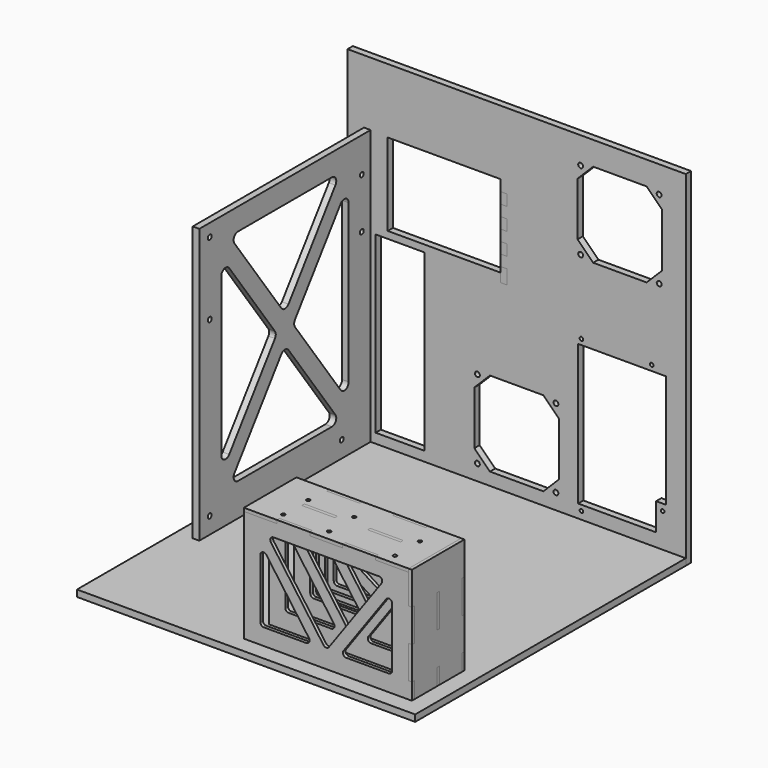
from build123d import *

# Parameters (mm, degrees)
F1_DEPTH  = 6
F3_DEPTH  = 6
F7_DEPTH  = 6
F10_D     = 4.4
F11_R     = 5
F12_W     = 44.5
F12_H     = 159
F12_W_2   = 102.7
F12_H_2   = 74.93
F13_DEPTH = 314.001
F15_W     = 22
F15_H     = 82.93
F16_DEPTH = 6
F17_W     = 6
F17_H     = 10
F18_DEPTH = 145.301
F21_DEPTH = 314.001
F22_D     = 3.3
F24_DEPTH = 314.001
F25_D     = 4.4
F27_W     = 153
F27_H     = 111
F28_DEPTH = 3
F29_W     = 30
F29_H     = 6
F29_H_2   = 3
F29_W_2   = 3
F29_H_3   = 30
F30_DEPTH = 315.001
F31_R     = 3
F35_W     = 150
F35_H     = 59.8
F36_DEPTH = 3
F38_D     = 3.3
F39_W     = 59.8
F39_H     = 105
F40_DEPTH = 3
F43_W     = 103
F43_H     = 79
F44_DEPTH = 3
F45_W     = 20
F45_H     = 6
F45_W_2   = 3
F45_H_2   = 2
F45_H_3   = 13
F45_H_4   = 3
F45_H_5   = 15
F46_DEPTH = 87.801
F47_R     = 3
F50_W     = 100
F50_H     = 23
F51_DEPTH = 3
F52_D     = 3.3
F55_W     = 23
F55_H     = 73
F56_DEPTH = 3


with BuildPart() as f1:
    # F0 (on Top) → F1 (new body)
    with BuildSketch(Plane.XY):
        Polygon((0, 314), (0, 0), (308, 0), (308, 308), (280, 308), (280, 314), (240, 314), (240, 308), (200, 308), (200, 314), (160, 314), (160, 308), (120, 308), (120, 314), (80, 314), (80, 308), (40, 308), (40, 314), align=None)
    extrude(amount=F1_DEPTH)


with BuildPart() as f3:
    # F2 (on face) → F3 (new body)
    with BuildSketch(Plane(origin=(0, 314, 0), x_dir=(-1, 0, 0), z_dir=(0, 1, 0))):
        Polygon((-308, 0), (-40, 0), (-40, 6), (0, 6), (0, 314), (-308, 314), align=None)
    extrude(amount=-F3_DEPTH)

    # F4: cut F1
    add(f1.part, mode=Mode.SUBTRACT)


with BuildPart() as f7:
    # F6 (on offset) → F7 (new body)
    with BuildSketch(Plane(origin=(15, 0, 0), x_dir=(0, -1, 0), z_dir=(-1, 0, 0))):
        Polygon((-284, 6), (-284, 0), (-254, 0), (-254, 6), (-224, 6), (-224, 0), (-194, 0), (-194, 6), (-164, 6), (-164, 0), (-134, 0), (-134, 6), (-113, 6), (-113, 256), (-308, 256), (-308, 246), (-314, 246), (-314, 216), (-308, 216), (-308, 186), (-314, 186), (-314, 156), (-308, 156), (-308, 126), (-314, 126), (-314, 96), (-308, 96), (-308, 66), (-314, 66), (-314, 36), (-308, 36), (-308, 6), align=None)
        Polygon((-210.5, 123.2224627651), (-147.2637144953, 36), (-273.7362855047, 36), align=None, mode=Mode.SUBTRACT)
        Polygon((-283, 48.7775372349), (-283, 223.2224627651), (-219.7637144953, 136), align=None, mode=Mode.SUBTRACT)
        Polygon((-201.2362855047, 136), (-138, 223.2224627651), (-138, 48.7775372349), align=None, mode=Mode.SUBTRACT)
        Polygon((-273.7362855047, 236), (-147.2637144953, 236), (-210.5, 148.7775372349), align=None, mode=Mode.SUBTRACT)
    extrude(amount=-F7_DEPTH)


with BuildPart() as f3_1:
    add(f3.part)

    # F8: cut F7
    add(f7.part, mode=Mode.SUBTRACT)

    # F12 (on face) → F13 (cut, through all)
    with BuildSketch(Plane(origin=(0, 314, 0), x_dir=(-1, 0, 0), z_dir=(0, 1, 0))):
        with Locations((-47.75, 94.3)):
            Rectangle(F12_W, F12_H)
        with Locations((-87.95, 217.615)):
            Rectangle(F12_W_2, F12_H_2)
    extrude(amount=-F13_DEPTH, mode=Mode.SUBTRACT)


with BuildPart() as f1_1:
    add(f1.part)

    # F9: cut F7
    add(f7.part, mode=Mode.SUBTRACT)


with BuildPart() as f7_1:
    add(f7.part)

    # F10 (through all)
    with Locations(Plane(origin=(15, 0, 0), x_dir=(0, -1, 0), z_dir=(-1, 0, 0))):
        with Locations((-298, 224.2), (-298, 178.48), (-275.14, 21), (-124.85, 21), (-124.85, 178.48), (-124.85, 244.52)):
            Hole(F10_D / 2)

    # F11
    f11_edges = [f7_1.edges().sort_by_distance(p)[0] for p in [
        (18, 283, 223.222463),
        (18, 210.5, 123.222463),
        (18, 147.263714, 36),
        (18, 138, 48.777537),
        (18, 201.236286, 136),
        (18, 138, 223.222463),
        (18, 147.263714, 236),
        (18, 210.5, 148.777537),
        (18, 219.763714, 136),
        (18, 283, 48.777537),
        (18, 273.736286, 36),
        (18, 273.736286, 236),
    ]]
    fillet(f11_edges, radius=F11_R)


with BuildPart() as f16:
    # F15 (on line) → F16 (new body)
    with BuildSketch(Plane(origin=(139.3, 0, 0), x_dir=(0, -1, 0), z_dir=(-1, 0, 0))):
        with Locations((-319, 213.615)):
            Rectangle(F15_W, F15_H)
    extrude(amount=-F16_DEPTH)

    # F17 (on face) → F18 (cut, through all)
    with BuildSketch(Plane.YZ.offset(145.3)):
        with Locations((311, 250.08)):
            Rectangle(F17_W, F17_H)
        with Locations((311, 230.08)):
            Rectangle(F17_W, F17_H)
        with Locations((311, 210.08)):
            Rectangle(F17_W, F17_H)
        with Locations((311, 190.08)):
            Rectangle(F17_W, F17_H)
    extrude(amount=-F18_DEPTH, mode=Mode.SUBTRACT)


with BuildPart() as f3_2:
    add(f3_1.part)

    # F19: cut F16
    add(f16.part, mode=Mode.SUBTRACT)

    # F20 (on face) → F21 (cut, through all)
    with BuildSketch(Plane(origin=(0, 314, 0), x_dir=(-1, 0, 0), z_dir=(0, 1, 0))):
        Polygon((-210, 146), (-290, 146), (-290, 43), (-281, 43), (-281, 18), (-210, 18), align=None)
    extrude(amount=-F21_DEPTH, mode=Mode.SUBTRACT)

    # F22 (through all)
    with Locations(Plane(origin=(0, 314, 0), x_dir=(-1, 0, 0), z_dir=(0, 1, 0))):
        with Locations((-277, 151), (-287, 37), (-213, 13), (-213, 151)):
            Hole(F22_D / 2)

    # F23 (on face) → F24 (cut, through all)
    with BuildSketch(Plane(origin=(0, 314, 0), x_dir=(-1, 0, 0), z_dir=(0, 1, 0))):
        Polygon((-129.6421356237, 94.5), (-178.3578643763, 94.5), (-192.5, 80.3578643763), (-192.5, 31.6421356237), (-178.3578643763, 17.5), (-129.6421356237, 17.5), (-115.5, 31.6421356237), (-115.5, 80.3578643763), align=None)
        Polygon((-223.6421356237, 292.5), (-272.3578643763, 292.5), (-286.5, 278.3578643763), (-286.5, 229.6421356237), (-272.3578643763, 215.5), (-223.6421356237, 215.5), (-209.5, 229.6421356237), (-209.5, 278.3578643763), align=None)
    extrude(amount=-F24_DEPTH, mode=Mode.SUBTRACT)

    # F25 (through all)
    with Locations(Plane(origin=(0, 314, 0), x_dir=(-1, 0, 0), z_dir=(0, 1, 0))):
        with Locations((-189.75, 91.75), (-189.75, 20.25), (-118.25, 20.25), (-118.25, 91.75), (-212.25, 218.25), (-283.75, 218.25), (-283.75, 289.75), (-212.25, 289.75)):
            Hole(F25_D / 2)


with BuildPart() as f28:
    # F27 (on offset) → F28 (new body)
    with BuildSketch(Plane.XZ.offset(-15)):
        with Locations((216.5, 55.5)):
            Rectangle(F27_W, F27_H)
        Polygon((202.6897369911, 21), (155, 21), (155, 87.4265764644), align=None, mode=Mode.SUBTRACT)
        Polygon((227.3102630089, 21), (275, 87.4265764644), (275, 21), align=None, mode=Mode.SUBTRACT)
        Polygon((215, 21), (161.1551315044, 96), (268.8448684956, 96), align=None, mode=Mode.SUBTRACT)
    extrude(amount=-F28_DEPTH)

    # F29 (on face) → F30 (cut, through all)
    with BuildSketch(Plane.XZ.offset(-15)):
        with Locations((155, 3)):
            Rectangle(F29_W, F29_H)
        with Locations((217, 3)):
            Rectangle(F29_W, F29_H)
        with Locations((279, 3)):
            Rectangle(F29_W, F29_H)
        with Locations((155, 109.5)):
            Rectangle(F29_W, F29_H_2)
        with Locations((215, 109.5)):
            Rectangle(F29_W, F29_H_2)
        Polygon((293, 111), (290, 111), (290, 108), (290, 81), (293, 81), align=None)
        with Locations((275, 109.5)):
            Rectangle(F29_W, F29_H_2)
        with Locations((291.5, 36)):
            Rectangle(F29_W_2, F29_H_3)
    extrude(amount=-F30_DEPTH, mode=Mode.SUBTRACT)

    # F31
    f31_edges = [f28.edges().sort_by_distance(p)[0] for p in [
        (161.155132, 16.5, 96),
        (155, 16.5, 87.426576),
        (215, 16.5, 21),
        (202.689737, 16.5, 21),
        (155, 16.5, 21),
        (227.310263, 16.5, 21),
        (275, 16.5, 21),
        (275, 16.5, 87.426576),
        (268.844868, 16.5, 96),
    ]]
    fillet(f31_edges, radius=F31_R)


with BuildPart() as f32_1:
    # F32: copy of F28
    add(f28.part.moved(Location((0, 28.4, 0))))


with BuildPart() as f33_1:
    # F33: copy of F32_1
    add(f32_1.part.moved(Location((0, 28.4, 0))))


with BuildPart() as f1_2:
    add(f1_1.part)

    # F34: cut F28, F32_1, F33_1
    add(f28.part, mode=Mode.SUBTRACT)
    add(f32_1.part, mode=Mode.SUBTRACT)
    add(f33_1.part, mode=Mode.SUBTRACT)


with BuildPart() as f36:
    # F35 (on face) → F36 (new body)
    with BuildSketch(Plane.XY.offset(108)):
        with Locations((215, 44.9)):
            Rectangle(F35_W, F35_H)
    extrude(amount=F36_DEPTH)

    # F37: cut F28, F32_1, F33_1
    add(f28.part, mode=Mode.SUBTRACT)
    add(f32_1.part, mode=Mode.SUBTRACT)
    add(f33_1.part, mode=Mode.SUBTRACT)

    # F38 (through all)
    with Locations(Plane(origin=(0, 0, 108), x_dir=(1, 0, 0), z_dir=(0, 0, -1))):
        with Locations((168.5, -52.75), (168.5, -24.35), (210.1, -24.35), (210.1, -52.75), (270.1, -52.75), (270.1, -24.35)):
            Hole(F38_D / 2)


with BuildPart() as f40:
    # F39 (on face) → F40 (new body)
    with BuildSketch(Plane.YZ.offset(290)):
        with Locations((44.9, 58.5)):
            Rectangle(F39_W, F39_H)
    extrude(amount=F40_DEPTH)

    # F41: cut F28, F32_1, F33_1
    add(f28.part, mode=Mode.SUBTRACT)
    add(f32_1.part, mode=Mode.SUBTRACT)
    add(f33_1.part, mode=Mode.SUBTRACT)


with BuildPart() as f44:
    # F43 (on offset) → F44 (new body)
    with BuildSketch(Plane(origin=(0, 84.8, 0), x_dir=(-1, 0, 0), z_dir=(0, 1, 0))):
        with Locations((-191.5, 39.5)):
            Rectangle(F43_W, F43_H)
        Polygon((-159.2904173616, 69), (-233, 21.9324351827), (-233, 69), align=None, mode=Mode.SUBTRACT)
        Polygon((-223.7095826384, 16), (-150, 63.0675648173), (-150, 16), align=None, mode=Mode.SUBTRACT)
    extrude(amount=F44_DEPTH)

    # F45 (on face) → F46 (cut, through all)
    with BuildSketch(Plane(origin=(0, 87.8, 0), x_dir=(-1, 0, 0), z_dir=(0, 1, 0))):
        with Locations((-150, 3)):
            Rectangle(F45_W, F45_H)
        with Locations((-192, 3)):
            Rectangle(F45_W, F45_H)
        Polygon((-244, 0), (-224, 0), (-224, 6), (-240, 6), (-240, 4), (-243, 4), (-243, 6), (-244, 6), align=None)
        with Locations((-241.5, 5)):
            Rectangle(F45_W_2, F45_H_2)
        with Locations((-241.5, 12.5)):
            Rectangle(F45_W_2, F45_H_3)
        Polygon((-240, 79), (-243, 79), (-243, 64), (-240, 64), (-240, 76), align=None)
        with Locations((-230, 77.5)):
            Rectangle(F45_W, F45_H_4)
        with Locations((-241.5, 41.5)):
            Rectangle(F45_W_2, F45_H_5)
        with Locations((-150, 77.5)):
            Rectangle(F45_W, F45_H_4)
        with Locations((-190, 77.5)):
            Rectangle(F45_W, F45_H_4)
    extrude(amount=-F46_DEPTH, mode=Mode.SUBTRACT)

    # F47
    f47_edges = [f44.edges().sort_by_distance(p)[0] for p in [
        (233, 86.3, 69),
        (150, 86.3, 16),
        (150, 86.3, 63.067565),
        (233, 86.3, 21.932435),
        (159.290417, 86.3, 69),
        (223.709583, 86.3, 16),
    ]]
    fillet(f47_edges, radius=F47_R)


with BuildPart() as f48_1:
    # F48: copy of F44
    add(f44.part.moved(Location((0, 10, 0))))


with BuildPart() as f49_1:
    # F49: copy of F48_1
    add(f48_1.part.moved(Location((0, 10, 0))))


with BuildPart() as f51:
    # F50 (on face) → F51 (new body)
    with BuildSketch(Plane.XY.offset(76)):
        with Locations((190, 96.3)):
            Rectangle(F50_W, F50_H)
    extrude(amount=F51_DEPTH)

    # F52 (through all)
    with Locations(Plane(origin=(0, 0, 76), x_dir=(1, 0, 0), z_dir=(0, 0, -1))):
        with Locations((154, -90.8), (154, -100.8), (230.6, -90.8), (230.6, -100.8)):
            Hole(F52_D / 2)

    # F53: cut F48_1, F44, F49_1
    add(f48_1.part, mode=Mode.SUBTRACT)
    add(f44.part, mode=Mode.SUBTRACT)
    add(f49_1.part, mode=Mode.SUBTRACT)


with BuildPart() as f1_3:
    add(f1_2.part)

    # F54: cut F44, F48_1, F49_1
    add(f44.part, mode=Mode.SUBTRACT)
    add(f48_1.part, mode=Mode.SUBTRACT)
    add(f49_1.part, mode=Mode.SUBTRACT)


with BuildPart() as f56:
    # F55 (on face) → F56 (new body)
    with BuildSketch(Plane.YZ.offset(240)):
        with Locations((96.3, 42.5)):
            Rectangle(F55_W, F55_H)
    extrude(amount=F56_DEPTH)

    # F57: cut F44, F48_1, F49_1
    add(f44.part, mode=Mode.SUBTRACT)
    add(f48_1.part, mode=Mode.SUBTRACT)
    add(f49_1.part, mode=Mode.SUBTRACT)


solid = Compound([f7_1.part, f16.part, f3_2.part, f28.part, f32_1.part, f33_1.part, f36.part, f40.part, f44.part, f48_1.part, f49_1.part, f51.part, f1_3.part, f56.part])
